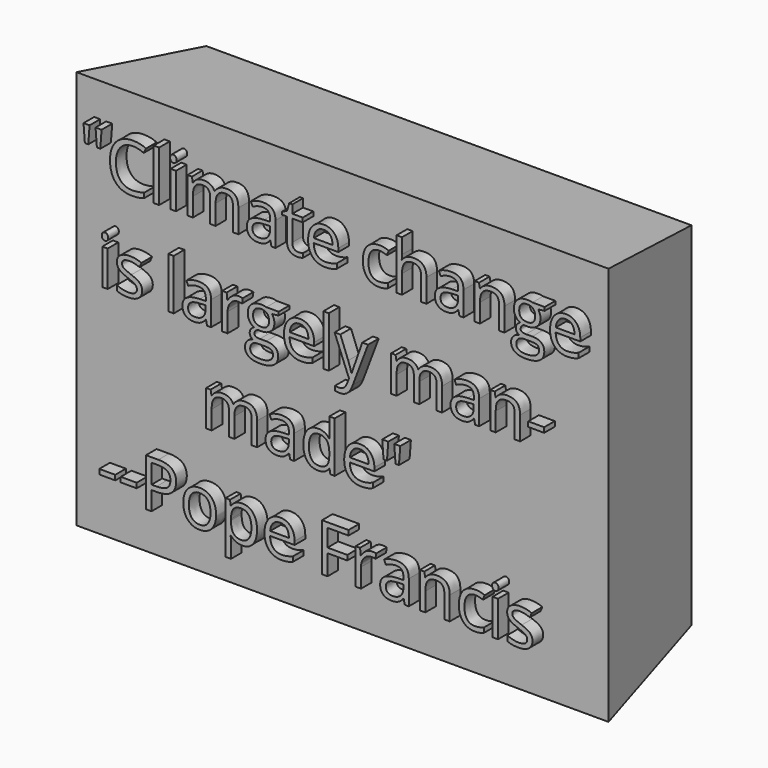
from build123d import *

# Parameters (mm, degrees)
F0_W         = 101.6
F0_H         = 76.2
F1_DEPTH     = 25.4
F1_TAPER     = 10
F2_TEXT_SIZE = 12.7350843195
F3_DEPTH     = 2.54


# Not quite as in the source:
# - Text() gives the source's letters only with a copy of the font that has no kerning and outlines rounded to 1/6400 em; it was checked with that copy


with BuildPart() as f1:
    # F0 (on Front) → F1 (new body)
    with BuildSketch(Plane.XZ):
        with Locations((-50.8, 38.1)):
            Rectangle(F0_W, F0_H)
    extrude(amount=-F1_DEPTH, taper=F1_TAPER)

    # F2 (on face) → F3 (join)
    with BuildSketch(Plane.XZ):
        with Locations((-99.06, 60.68073929)):
            Text('"Climate change', F2_TEXT_SIZE, font='Open Sans', text_align=(TextAlign.LEFT, TextAlign.BOTTOM))
        with Locations((-95.7508679339, 43.3610246155)):
            Text('is largely man-', F2_TEXT_SIZE, font='Open Sans', text_align=(TextAlign.LEFT, TextAlign.BOTTOM))
        with Locations((-75.896075537, 26.041309941)):
            Text('made"', F2_TEXT_SIZE, font='Open Sans', text_align=(TextAlign.LEFT, TextAlign.BOTTOM))
        with Locations((-95.7508679339, 8.7215952666)):
            Text('--Pope Francis', F2_TEXT_SIZE, font='Open Sans', text_align=(TextAlign.LEFT, TextAlign.BOTTOM))
    extrude(amount=F3_DEPTH)


solid = f1.part
